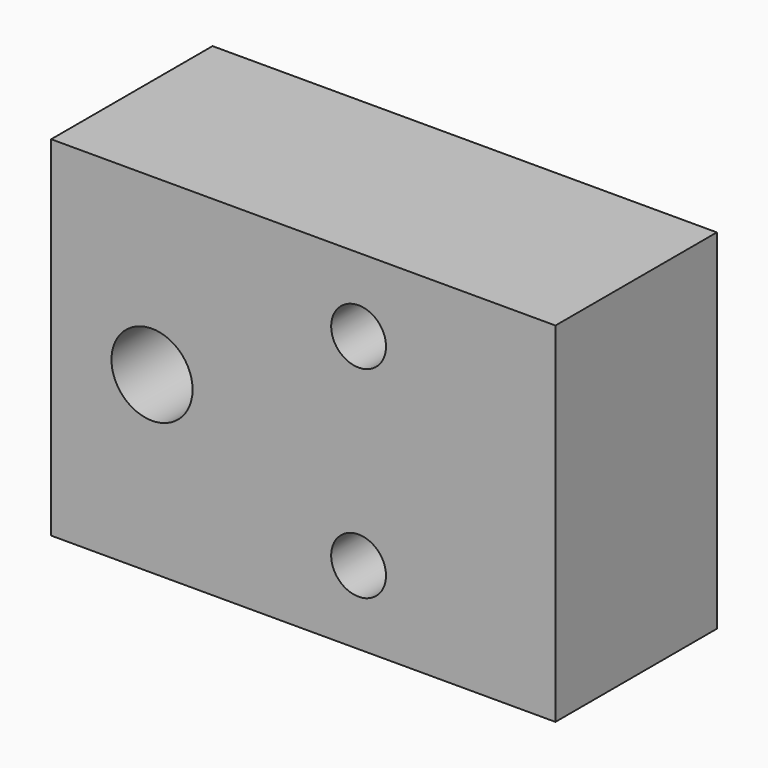
from build123d import *

# Parameters (mm, degrees)
F0_W     = 3.4798
F0_H     = 6.35
F0_W_2   = 12.3952
F1_DEPTH = 12.7
F2_D     = 3.4544
F4_D     = 5.1054


# Not quite as in the source:
# - a feature names something its author has since deleted; it is built from what else it names


with BuildPart() as f1:
    # F0 (on Front) → F1 (new body)
    with BuildSketch(Plane.XZ):
        Polygon((0, -6.35), (0, 0), (-15.875, 0), (-15.875, -10.9855), (0, -10.9855), align=None)
        Polygon((-15.875, 0), (0, 0), (0, 6.35), (0, 10.9855), (-15.875, 10.9855), align=None)
        Polygon((0, 10.9855), (0, 6.35), (3.4798, 6.35), (15.875, 6.35), (15.875, 10.9855), align=None)
        with Locations((1.7399, 3.175)):
            Rectangle(F0_W, F0_H)
        with Locations((9.6774, 3.175)):
            Rectangle(F0_W_2, F0_H)
        with Locations((9.6774, -3.175)):
            Rectangle(F0_W_2, F0_H)
        with Locations((1.7399, -3.175)):
            Rectangle(F0_W, F0_H)
        Polygon((3.4798, -6.35), (0, -6.35), (0, -10.9855), (15.875, -10.9855), (15.875, -6.35), align=None)
    extrude(amount=-F1_DEPTH)

    # F2 (through all)
    with Locations(Plane.XZ):
        with Locations((3.4798, -6.35), (3.4798, 6.35)):
            Hole(F2_D / 2)

    # F4 (through all)
    with Locations(Plane(origin=(0, 12.7, 0), x_dir=(-1, 0, 0), z_dir=(0, 1, 0))):
        with Locations((9.525, 0)):
            Hole(F4_D / 2)


solid = f1.part
